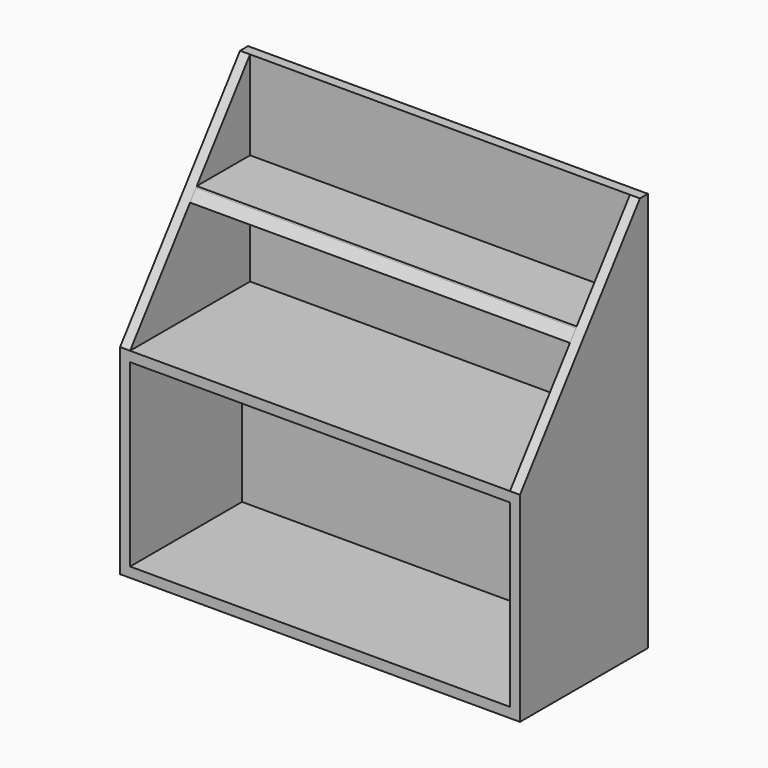
from build123d import *

# Parameters (mm, degrees)
F0_W      = 20
F0_H      = 8
F1_DEPTH  = 5
F2_W      = 20
F2_H      = 0.5
F3_DEPTH  = 10
F5_DEPTH  = 0.5
F7_DEPTH  = 0.5
F8_DEPTH  = 5
F11_W     = 19
F11_H     = 0.5570442975
F12_DEPTH = 4
F14_DEPTH = 25
F15_W     = 19
F15_H     = 9
F16_DEPTH = 7


# Not quite as in the source:
# - a feature of the source that left no trace in its solid (it failed there, or was rolled back) is left out


with BuildPart() as f1:
    # F0 (on Top) → F1 (new body)
    with BuildSketch(Plane.XY):
        with Locations((8.2929818355, 4)):
            Rectangle(F0_W, F0_H)
    extrude(amount=F1_DEPTH)

    # F2 (on face) → F3 (join)
    with BuildSketch(Plane.XY.offset(5)):
        with Locations((8.2929818355, 7.75)):
            Rectangle(F2_W, F2_H)
    extrude(amount=F3_DEPTH)

    # F4 (on face) → F5 (join)
    with BuildSketch(Plane(origin=(-1.7070181645, 0, 0), x_dir=(0, -1, 0), z_dir=(-1, 0, 0))):
        Polygon((-7.5, 5), (0, 5), (-7.5, 15), align=None)
    extrude(amount=-F5_DEPTH)

    # F6 (on face) → F7 (join)
    with BuildSketch(Plane.YZ.offset(18.2929818355)):
        Polygon((7.5, 5), (7.5, 15), (0, 5), align=None)
    extrude(amount=-F7_DEPTH)

    # F8 (add): a face of the model
    f8_faces = [f1.faces().sort_by_distance(p)[0] for p in [
        (8.2929818355, 4, 0),
    ]]
    extrude(f8_faces, amount=F8_DEPTH)

    # F11 (on face) → F12 (join)
    with BuildSketch(Plane.XZ.offset(-7.5)):
        with Locations((8.2929818355, 10.2785221487)):
            Rectangle(F11_W, F11_H)
    extrude(amount=F12_DEPTH)

    # F13 (on face) → F14 (cut)
    with BuildSketch(Plane.YZ.offset(17.7929818355)):
        Polygon((3.75, 10), (4.1247227065, 10.4996302754), (4.1677832231, 10.5570442975), (3.5, 10.5570442975), (3.5, 10), align=None)
    extrude(amount=-F14_DEPTH, mode=Mode.SUBTRACT)

    # F15 (on face) → F16 (cut)
    with BuildSketch(Plane.XZ):
        with Locations((8.2929818355, 0)):
            Rectangle(F15_W, F15_H)
    extrude(amount=-F16_DEPTH, mode=Mode.SUBTRACT)


solid = f1.part
